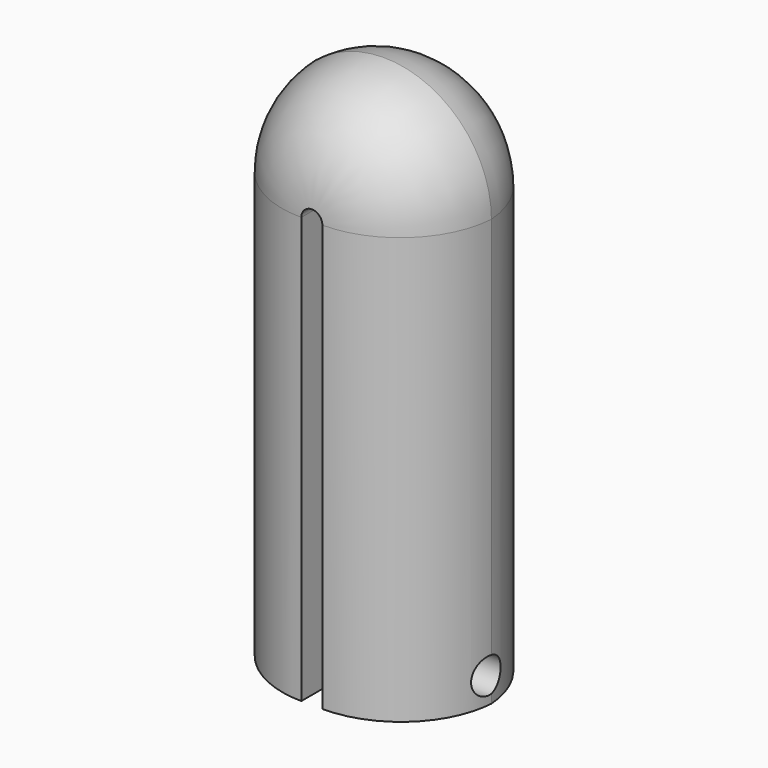
from build123d import *

# Parameters (mm, degrees)
F1_DEPTH    = 33.02
F2_T1_DEPTH = 122.514239143
F2_T3_DEPTH = 122.3049164534
F2_T6_ANGLE = 180
F2_T8_ANGLE = 180
F3_DEPTH    = 127
F5_D        = 6.35
F5_DEPTH    = 19.6628549222
F6_D        = 6.35


# Not quite as in the source:
# - a fillet or chamfer that OpenCascade refuses, or shapes differently, is made with other operations: its cross-section is extruded or revolved along the edge and cut away or added


with BuildPart() as f1:
    # F0 (on Front) → F1 (new body)
    with BuildSketch(Plane.XZ):
        with BuildLine():
            Line((-19.7072699666, 0), (19.7072699666, 0))
            ThreePointArc((19.7072699666, 0), (0, 19.7072699666), (-19.7072699666, 0))
        make_face()
        Polygon((19.7072699666, -78.064239143), (19.7072699666, 0), (-19.7072699666, 0), (-19.7072699666, -77.8549164534), align=None)
    extrude(amount=F1_DEPTH)

    # F2: fillet of radius 17.78 on 2 edges, made by hand

    # F2_s2 → F2_t1 (cut)
    with BuildSketch(Plane.XY.offset(-122.514239143)):
        with BuildLine():
            ThreePointArc((19.7072699666, -17.78), (14.4996285361, -5.2076414305), (1.9272699666, 0))
            Line((1.9272699666, 0), (19.7072699666, 0))
            Line((19.7072699666, 0), (19.7072699666, -17.78))
        make_face()
        with BuildLine():
            ThreePointArc((19.7072699666, -15.24), (14.4996285361, -27.8123585695), (1.9272699666, -33.02))
            Line((1.9272699666, -33.02), (19.7072699666, -33.02))
            Line((19.7072699666, -33.02), (19.7072699666, -15.24))
        make_face()
    extrude(amount=F2_T1_DEPTH, mode=Mode.SUBTRACT)

    # F2_s4 → F2_t3 (cut)
    with BuildSketch(Plane.XY.offset(-122.3049164534)):
        with BuildLine():
            ThreePointArc((-19.7072699666, -15.24), (-14.4996285361, -27.8123585695), (-1.9272699666, -33.02))
            Line((-1.9272699666, -33.02), (-19.7072699666, -33.02))
            Line((-19.7072699666, -33.02), (-19.7072699666, -15.24))
        make_face()
        with BuildLine():
            ThreePointArc((-19.7072699666, -17.78), (-14.4996285361, -5.2076414305), (-1.9272699666, 0))
            Line((-1.9272699666, 0), (-19.7072699666, 0))
            Line((-19.7072699666, 0), (-19.7072699666, -17.78))
        make_face()
    extrude(amount=F2_T3_DEPTH, mode=Mode.SUBTRACT)

    # F2_s5 → F2_t6 (revolve, cut)
    with BuildSketch(Plane.XY):
        with BuildLine():
            ThreePointArc((19.7072699666, -15.24), (14.4996285361, -27.8123585695), (1.9272699666, -33.02))
            Line((1.9272699666, -33.02), (19.7072699666, -33.02))
            Line((19.7072699666, -33.02), (19.7072699666, -15.24))
        make_face()
    revolve(axis=Axis((0, -33.02, 0), (0, -1, 0)), revolution_arc=F2_T6_ANGLE, mode=Mode.SUBTRACT)

    # F2_s7 → F2_t8 (revolve, cut)
    with BuildSketch(Plane.XY):
        with BuildLine():
            ThreePointArc((19.7072699666, -17.78), (14.4996285361, -5.2076414305), (1.9272699666, 0))
            Line((1.9272699666, 0), (19.7072699666, 0))
            Line((19.7072699666, 0), (19.7072699666, -17.78))
        make_face()
    revolve(axis=Axis((0, 0, 0), (0, -1, 0)), revolution_arc=F2_T8_ANGLE, mode=Mode.SUBTRACT)

    # F3 (cut): a face of the model
    f3_faces = [f1.faces().sort_by_distance(p)[0] for p in [
        (8.27376e-05, -33.02, -38.2217878295),
    ]]
    extrude(f3_faces, amount=-F3_DEPTH, mode=Mode.SUBTRACT)

    # F5 (through all, one way)
    with BuildSketch(Plane.YZ):
        with Locations((-17.1199291945, -73.3298659325)):
            Circle(F5_D / 2)
    extrude(amount=-F5_DEPTH, mode=Mode.SUBTRACT)

    # F6 (through all)
    with Locations(Plane(origin=(0, 0, 0), x_dir=(0, 1, 0), z_dir=(-1, 0, 0))):
        with Locations((-17.1199291945, 73.3298659325)):
            Hole(F6_D / 2)


solid = f1.part
